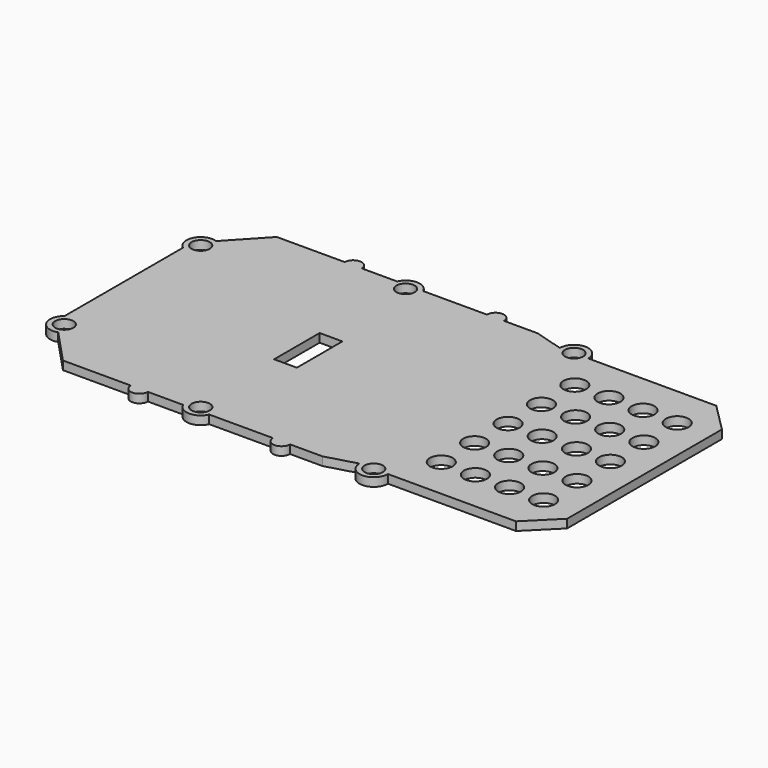
from build123d import *

# Parameters (mm, degrees)
F0_R     = 1.6
F0_W     = 4
F0_H     = 10
F0_R_2   = 2
F1_DEPTH = 1.5


# Not quite as in the source:
# - ends of sketch curves that miss each other by under 0.0002 mm in the source are joined


with BuildPart() as f1:
    # F0 (on Top) → F1 (new body)
    with BuildSketch(Plane.XY):
        with BuildLine():
            Line((25.1510733024, -23.3822189373), (30.8373828109, -23.3822189373))
            Line((30.8373828109, -23.3822189373), (36.1510733024, -21.8822189373))
            ThreePointArc((36.1510733024, -21.8822189373), (38.6560733124, -24.3822139373), (41.1510533024, -21.8722189373))
            Line((41.1510533024, -21.8722189373), (63.6510733024, -21.8722189373))
            Line((63.6510733024, -21.8722189373), (68.6510733024, -16.8822189373))
            Line((68.6510733024, -16.8822189373), (68.6510733024, 17.1177810627))
            Line((68.6510733024, 17.1177810627), (63.6510733024, 22.1277810627))
            Line((63.6510733024, 22.1277810627), (41.1510733024, 22.1277810627))
            ThreePointArc((41.1510733024, 22.1277810627), (38.6510733024, 24.6277810627), (36.1510733024, 22.1277810627))
            Line((36.1510733024, 22.1277810627), (31.0856380889, 23.6277810627))
            Line((31.0856380889, 23.6277810627), (25.1510399687, 23.6277810627))
            ThreePointArc((25.1510399687, 23.6277810627), (23.6460732747, 25.1177727292), (22.1510733024, 23.6177810627))
            Line((22.1510733024, 23.6177810627), (10.9423611499, 23.6177810627))
            ThreePointArc((10.9423611499, 23.6177810627), (8.6510733024, 25.1177810627), (6.359785455, 23.6177810627))
            Line((6.359785455, 23.6177810627), (0.1508824054, 23.6177810627))
            ThreePointArc((0.1508824054, 23.6177810627), (-1.3489266976, 25.0938508558), (-2.8487358005, 23.6177810627))
            Line((-2.8487358005, 23.6177810627), (-14.783491484, 23.6177810627))
            Line((-14.783491484, 23.6177810627), (-20.5213222757, 17.4701052144))
            ThreePointArc((-20.5213222757, 17.4701052144), (-23.5739450953, 16.2938104546), (-22.8489266976, 13.1037440347))
            Line((-22.8489266976, 13.1037440347), (-22.8489266976, -12.9160506452))
            ThreePointArc((-22.8489266976, -12.9160506452), (-23.5205541523, -16.0850132599), (-20.5005032054, -17.2566359677))
            Line((-20.5005032054, -17.2566359677), (-14.7737467559, -23.3822189373))
            Line((-14.7737467559, -23.3822189373), (-2.8489266976, -23.3822189373))
            ThreePointArc((-2.8489266976, -23.3822189373), (-1.3489266976, -24.8822189373), (0.1510733024, -23.3822189373))
            Line((0.1510733024, -23.3822189373), (6.359785455, -23.3822189373))
            ThreePointArc((6.359785455, -23.3822189373), (8.6510733024, -24.8822189373), (10.9423611499, -23.3822189373))
            Line((10.9423611499, -23.3822189373), (22.1510733024, -23.3822189373))
            ThreePointArc((22.1510733024, -23.3822189373), (23.6510729001, -24.8822181327), (25.1510733024, -23.3822189373))
        make_face()
        with Locations((-21.3217459931, -14.8953735334)):
            Circle(F0_R, mode=Mode.SUBTRACT)
        with Locations((8.6510733024, -22.3822189373)):
            Circle(F0_R, mode=Mode.SUBTRACT)
        with Locations((9.6388893649, 1.118e-07)):
            Rectangle(F0_W, F0_H, mode=Mode.SUBTRACT)
        with Locations((38.6510733024, -21.8822189373)):
            Circle(F0_R, mode=Mode.SUBTRACT)
        with Locations((44.6510733024, -14.5422189373)):
            Circle(F0_R_2, mode=Mode.SUBTRACT)
        with Locations((50.6510733024, -14.5422189373)):
            Circle(F0_R_2, mode=Mode.SUBTRACT)
        with Locations((56.6510733024, -14.5422189373)):
            Circle(F0_R_2, mode=Mode.SUBTRACT)
        with Locations((62.6510733024, -14.5422189373)):
            Circle(F0_R_2, mode=Mode.SUBTRACT)
        with Locations((44.6510733024, -7.2122189373)):
            Circle(F0_R_2, mode=Mode.SUBTRACT)
        with Locations((50.6510733024, -7.2122189373)):
            Circle(F0_R_2, mode=Mode.SUBTRACT)
        with Locations((56.6510733024, -7.2122189373)):
            Circle(F0_R_2, mode=Mode.SUBTRACT)
        with Locations((62.6510733024, -7.2122189373)):
            Circle(F0_R_2, mode=Mode.SUBTRACT)
        with Locations((-21.3678274943, 15.1177810627)):
            Circle(F0_R, mode=Mode.SUBTRACT)
        with Locations((8.6510733024, 22.6177810627)):
            Circle(F0_R, mode=Mode.SUBTRACT)
        with Locations((44.6510733024, 0.1277810627)):
            Circle(F0_R_2, mode=Mode.SUBTRACT)
        with Locations((44.6510733024, 7.4677810627)):
            Circle(F0_R_2, mode=Mode.SUBTRACT)
        with Locations((50.6510733024, 0.1277810627)):
            Circle(F0_R_2, mode=Mode.SUBTRACT)
        with Locations((56.6822756082, 0.1277810627)):
            Circle(F0_R_2, mode=Mode.SUBTRACT)
        with Locations((62.6510733024, 0.1277810627)):
            Circle(F0_R_2, mode=Mode.SUBTRACT)
        with Locations((50.6510733024, 7.4677810627)):
            Circle(F0_R_2, mode=Mode.SUBTRACT)
        with Locations((56.6510733024, 7.4677810627)):
            Circle(F0_R_2, mode=Mode.SUBTRACT)
        with Locations((62.6510733024, 7.4677810627)):
            Circle(F0_R_2, mode=Mode.SUBTRACT)
        with Locations((44.6510733024, 14.7977810627)):
            Circle(F0_R_2, mode=Mode.SUBTRACT)
        with Locations((38.6510733024, 22.1277810627)):
            Circle(F0_R, mode=Mode.SUBTRACT)
        with Locations((50.6510733024, 14.7977810627)):
            Circle(F0_R_2, mode=Mode.SUBTRACT)
        with Locations((56.6510733024, 14.7977810627)):
            Circle(F0_R_2, mode=Mode.SUBTRACT)
        with Locations((62.6510733024, 14.7977810627)):
            Circle(F0_R_2, mode=Mode.SUBTRACT)
    extrude(amount=F1_DEPTH)


solid = f1.part
